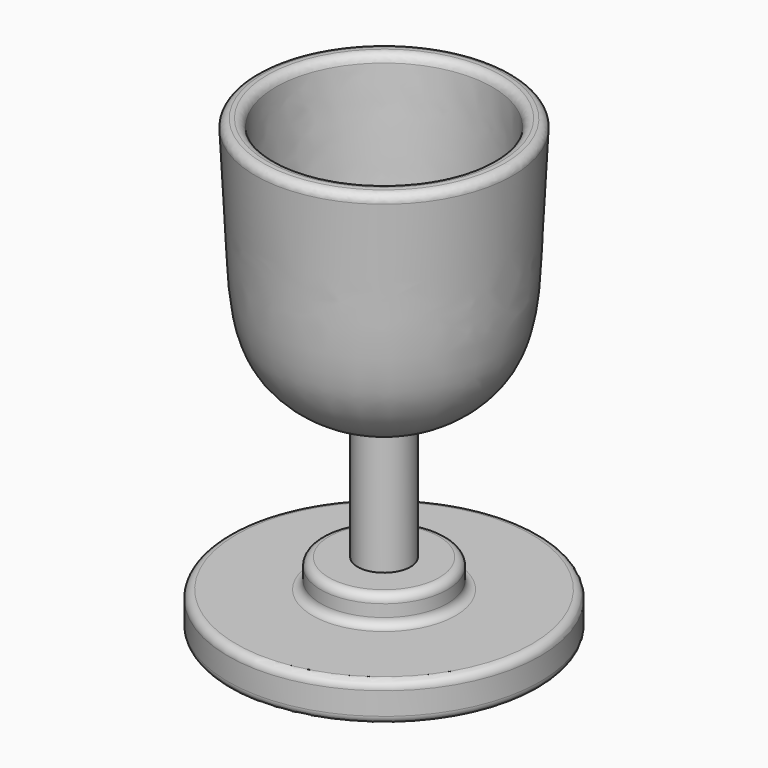
from build123d import *

# Parameters (mm, degrees)
F2_R = 2.54


# Not quite as in the source:
# - ends of sketch curves that miss each other by under 0.0002 mm in the source are joined
# - the dataset's text gives a spline's control points without its knots; the knots are read off the source's solid


with BuildPart() as f1:
    # F0 (on Front) → F1 (revolve)
    with BuildSketch(Plane.XZ):
        with BuildLine():
            Line((0, 68.2004094124), (0, 0))
            Line((0, 0), (48.7145781517, 0))
            Line((48.7145781517, 0), (48.7145781517, 12.1048344299))
            Line((48.7145781517, 12.1048344299), (19.7810716927, 12.1048344299))
            Line((19.7810716927, 12.1048344299), (19.7810716927, 20.9620315582))
            Line((19.7810716927, 20.9620315582), (8.2667153329, 20.9620315582))
            Line((8.2667153329, 20.9620315582), (8.2667153329, 61.7529523352))
            add(Edge.make_bspline(
                [(8.2667153329, 61.7529523352), (8.2888330219, 61.7495596613), (8.8211284351, 61.6707183939), (9.7579637458, 61.5668484345), (11.1620979745, 61.5709071244), (12.2801866906, 61.6606702124), (13.4367149147, 61.8449502056), (14.6253409937, 62.1282765472), (15.7942388523, 62.4916061819), (17.3533276727, 63.07316192), (19.3278629535, 63.9785150936), (21.7486186571, 65.3473415088), (24.1878759778, 67.0019438004), (26.5962424637, 68.9487958984), (28.5269316204, 70.8241749795), (29.9895556674, 72.4845402431), (30.861047091, 73.5915011756), (31.5263889999, 74.5189641679), (32.1702335281, 75.4779615602), (32.9121217451, 76.7052047107), (33.7053218967, 78.2118173229), (34.6423947788, 80.2582249193), (35.6044653938, 82.871665416), (36.4806441667, 86.0647574631), (37.3484454906, 90.3723702932), (37.8628296757, 94.7285765961), (38.1833195214, 99.0872514908), (38.3601364772, 102.3448248374), (38.4811168094, 105.0365585084), (38.5776258479, 107.1705077909), (38.6761556925, 109.3126007804), (38.8020494714, 111.997252289), (39.0090811236, 116.3092930912), (39.2770612873, 121.7258371812), (39.6097551265, 128.2585688128), (39.9499057112, 134.8141032569), (40.1792137513, 139.1930706481), (40.2938940846, 141.3830564792)],
                knots=[0.0298831344, 0.0298831344, 0.0298831344, 0.0298831344, 0.03125, 0.0625, 0.078125, 0.09375, 0.109375, 0.125, 0.140625, 0.15625, 0.1875, 0.21875, 0.25, 0.28125, 0.3125, 0.328125, 0.34375, 0.3515625, 0.359375, 0.375, 0.390625, 0.40625, 0.4375, 0.46875, 0.5, 0.5625, 0.59375, 0.625, 0.65625, 0.671875, 0.6875, 0.71875, 0.75, 0.8125, 0.875, 0.9375, 1, 1, 1, 1], degree=3))
            Line((40.2938940846, 141.3830564792), (33.9525826275, 141.7151242495))
            add(Edge.make_bspline(
                [(8.2667153329, 68.2004094124), (9.5223581478, 67.9597205701), (13.2598220275, 67.2433019806), (31.0143168645, 77.7500606958), (32.1499123228, 107.2905432418), (33.3295559895, 129.8175349272), (33.9525826275, 141.7151242495)],
                knots=[0, 0, 0, 0, 0.1199724945, 0.3571022422, 0.6604547289, 1, 1, 1, 1], degree=3))
            Line((8.2667153329, 68.2004094124), (0, 68.2004094124))
        make_face()
    revolve(axis=Axis((0, 0, 34.1002047062), (0, 0, -1)))

    # F2
    f2_edges = [f1.edges().sort_by_distance(p)[0] for p in [
        (-19.781072, 0, 20.962032),
        (-48.714578, 0, 12.104834),
        (-33.952583, 0, 141.715124),
        (-19.781072, 0, 12.104834),
        (-48.714578, 0, 0),
        (-40.293894, 0, 141.383056),
    ]]
    fillet(f2_edges, radius=F2_R)


solid = f1.part
